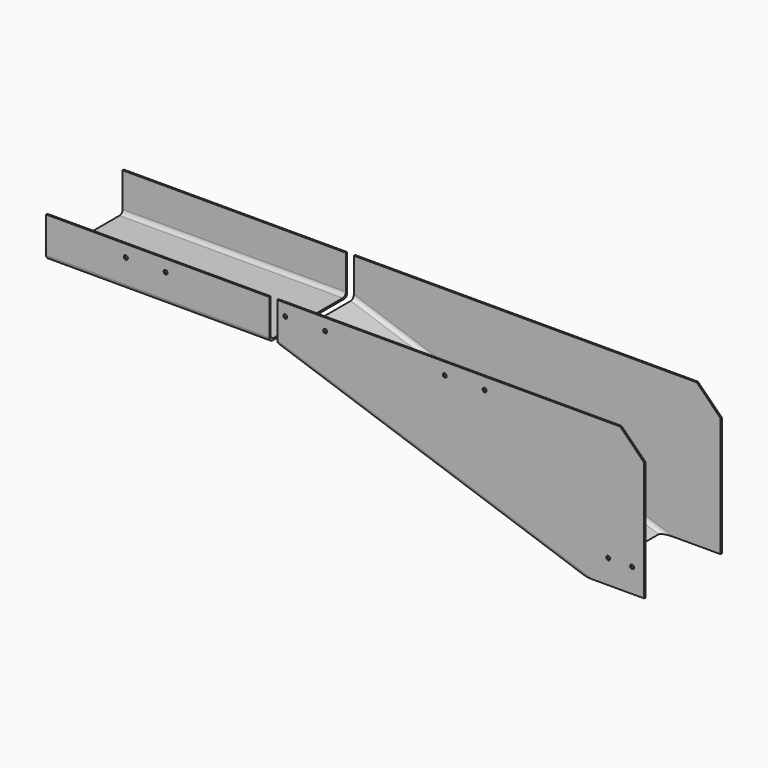
from build123d import *

# Parameters (mm, degrees)
F1_DEPTH = 122
F2_T     = -2
F3_R     = 5
F4_SIZE  = 30
F5_W     = 280
F5_H     = 50
F6_DEPTH = 122
F7_T     = -2
F8_R     = 2.5
F9_DEPTH = 25
F10_R    = 5


with BuildPart() as f1:
    # F0 (on Front) → F1 (new body)
    with BuildSketch(Plane.XZ):
        Polygon((-80, 0), (0, 0), (0, 180), (-460, 180), (-460, 130), align=None)
    extrude(amount=-F1_DEPTH)

    # F2
    f2_openings = [f1.faces().sort_by_distance(p)[0] for p in [
        (-230, 61, 180),
        (0, 61, 90),
        (-40, 61, 0),
        (-460, 61, 155),
    ]]
    offset(amount=F2_T, openings=f2_openings)

    # F3
    f3_edges = [f1.edges().sort_by_distance(p)[0] for p in [
        (-270, 0, 65),
        (-270, 122, 65),
        (-266.910602, 2, 66.056899),
        (-266.910602, 120, 66.056899),
    ]]
    fillet(f3_edges, radius=F3_R)

    # F4
    f4_edges = [f1.edges().sort_by_distance(p)[0] for p in [
        (0, 1, 180),
        (0, 121, 180),
    ]]
    chamfer(f4_edges, length=F4_SIZE)


with BuildPart() as f6:
    # F5 (on Front) → F6 (new body)
    with BuildSketch(Plane.XZ):
        with Locations((-610, 155)):
            Rectangle(F5_W, F5_H)
    extrude(amount=-F6_DEPTH)

    # F7
    f7_openings = [f6.faces().sort_by_distance(p)[0] for p in [
        (-610, 61, 180),
        (-470, 61, 155),
        (-750, 61, 155),
    ]]
    offset(amount=F7_T, openings=f7_openings)


with BuildPart() as f9_tool:
    # F8 (on face) → F9 (new body)
    with BuildSketch(Plane.XZ):
        with Locations((-45, 30)):
            Circle(F8_R)
        with Locations((-15, 30)):
            Circle(F8_R)
        with Locations((-450, 165)):
            Circle(F8_R)
        with Locations((-400, 165)):
            Circle(F8_R)
        with Locations((-250, 165)):
            Circle(F8_R)
        with Locations((-200, 165)):
            Circle(F8_R)
        with Locations((-650, 165)):
            Circle(F8_R)
        with Locations((-600, 165)):
            Circle(F8_R)
    extrude(amount=-F9_DEPTH)


with BuildPart() as f1_1:
    add(f1.part)

    # F9: cut by f9_tool
    add(f9_tool.part, mode=Mode.SUBTRACT)


with BuildPart() as f6_1:
    add(f6.part)

    # F9: cut by f9_tool
    add(f9_tool.part, mode=Mode.SUBTRACT)

    # F10
    f10_edges = [f6_1.edges().sort_by_distance(p)[0] for p in [
        (-610, 0, 130),
        (-610, 122, 130),
        (-610, 120, 132),
        (-610, 2, 132),
    ]]
    fillet(f10_edges, radius=F10_R)


solid = Compound([f1_1.part, f6_1.part])
